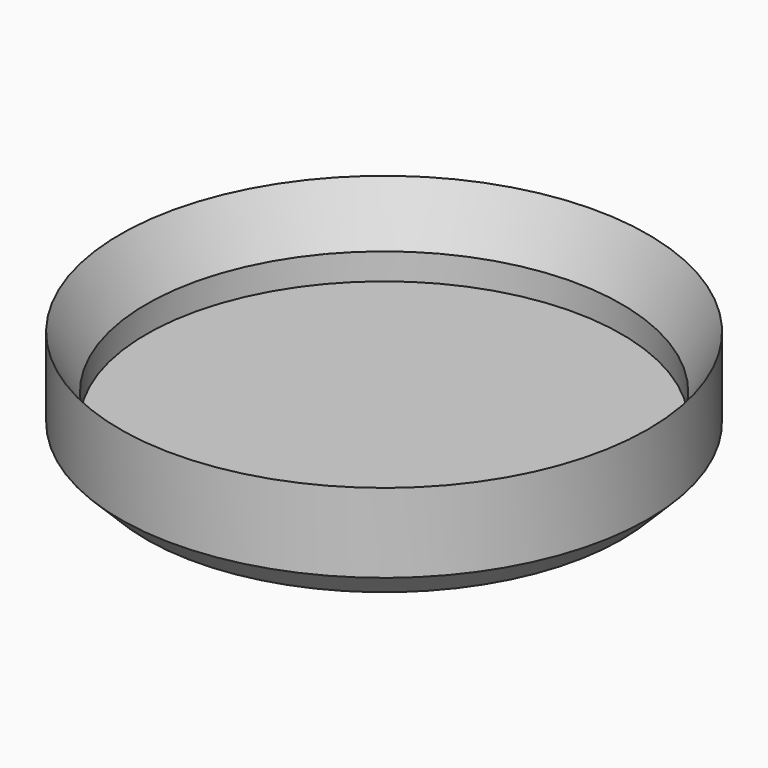
from build123d import *

# Parameters (mm, degrees)
F0_R     = 45
F1_DEPTH = 5
F0_R_2   = 50
F2_DEPTH = 20
F3_SIZE2 = 5
F3_SIZE  = 5
F4_SIZE2 = 4.99999
F4_SIZE  = 9.99999


# Not quite as in the source:
# - a fillet or chamfer is up to 0.001 mm smaller than in the source, because OpenCascade refuses the exact size
# - a feature of the source that left no trace in its solid (it failed there, or was rolled back) is left out


with BuildPart() as f1:
    # F0 (on Top) → F1 (new body)
    with BuildSketch(Plane.XY):
        Circle(F0_R)
    extrude(amount=F1_DEPTH)

    # F0 (on Top) → F2 (join)
    with BuildSketch(Plane.XY):
        Circle(F0_R_2)
        Circle(F0_R, mode=Mode.SUBTRACT)
    extrude(amount=F2_DEPTH)

    # F3
    f3_edges = [f1.edges().sort_by_distance(p)[0] for p in [
        (-50, 0, 0),
    ]]
    chamfer(f3_edges, length=F3_SIZE, length2=F3_SIZE2)

    # F4 (size 10 and 5 in the source; OpenCascade refuses exactly that, so slightly less here)
    f4_edges = [f1.edges().sort_by_distance(p)[0] for p in [
        (-45, 0, 20),
    ]]
    f4_side = f1.faces().sort_by_distance((-45, 0, 12.5))[0]
    chamfer(f4_edges, length=F4_SIZE, length2=F4_SIZE2, reference=f4_side)


solid = f1.part
